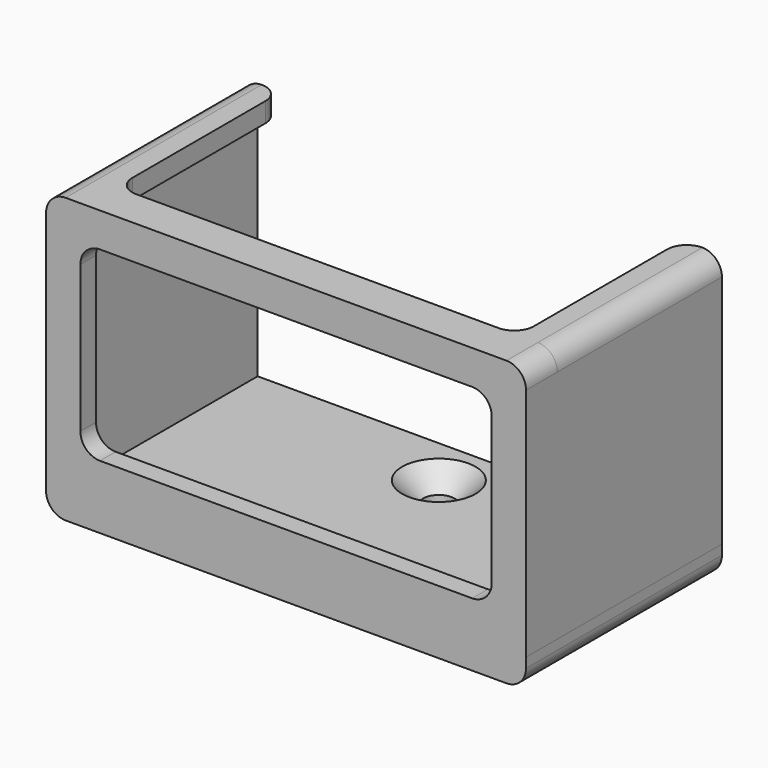
from build123d import *

# Parameters (mm, degrees)
F1_DEPTH        = 24
F2_W            = 4
F2_H            = 21
F3_DEPTH        = 2
F4_W            = 42
F4_H            = 19
F5_DEPTH        = 25
F6_W            = 48.9999982978
F6_H            = 25
F7_DEPTH        = 3
F8_F1_R         = 2
F8_F2_R         = 2
F8_F3_R         = 1.9999
F8_F4_R         = 1.9999
F8_F5_R         = 2
F8_F6_R         = 2
F8_F7_R         = 2
F8_F8_R         = 2
F8_F9_R         = 2
F8_F10_R        = 2
F8_F11_R        = 2
F8_F12_R        = 2
F10_D           = 3.2
F10_CSINK_D     = 7.5
F10_CSINK_ANGLE = 90
F11_R           = 1
F12_SIZE        = 0.5


# Not quite as in the source:
# - a fillet or chamfer is up to 0.001 mm smaller than in the source, because OpenCascade refuses the exact size
# - ends of sketch curves that miss each other by under 0.0002 mm in the source are joined


with BuildPart() as f1:
    # F0 (on Top) → F1 (new body)
    with BuildSketch(Plane.XY):
        Polygon((22.499999217, -11.5), (-22.500000783, -11.5), (-22.499999217, 11.5), (-24.499999217, 11.5), (-24.5000009192, -13.5), (24.4999990808, -13.5), (24.500000783, 11.5), (22.500000783, 11.5), align=None)
    extrude(amount=F1_DEPTH)

    # F2 (on face) → F3 (join)
    with BuildSketch(Plane.XY.offset(24)):
        Polygon((-24.5000009192, -9.5), (-24.5000009192, -13.5), (24.4999993532, -13.5), (24.4999993532, -9.5), (20.500000783, -9.5), (-20.499999217, -9.5), align=None)
        with Locations((-22.499999217, 1)):
            Rectangle(F2_W, F2_H)
        Polygon((20.500000783, -9.5), (24.4999993532, -9.5), (24.500000783, 11.5), (20.500000783, 11.5), align=None)
    extrude(amount=F3_DEPTH)

    # F4 (on face) → F5 (cut)
    with BuildSketch(Plane.XZ.offset(13.5)):
        with Locations((-9.192e-07, 13)):
            Rectangle(F4_W, F4_H)
    extrude(amount=-F5_DEPTH, mode=Mode.SUBTRACT)

    # F6 (on face) → F7 (join)
    with BuildSketch(Plane(origin=(0, 0, 0), x_dir=(1, 0, 0), z_dir=(0, 0, -1))):
        with Locations((-6.81e-08, 1)):
            Rectangle(F6_W, F6_H)
    extrude(amount=F7_DEPTH)

    # F8: fillet of radius 2 on 14 edges, made by hand

    # F8_f1
    f8_f1_edges = [f1.edges().sort_by_distance(p)[0] for p in [
        (20.500000783, 11.5, 25),
    ]]
    fillet(f8_f1_edges, radius=F8_F1_R)

    # F8_f2
    f8_f2_edges = [f1.edges().sort_by_distance(p)[0] for p in [
        (-20.499999217, 11.5, 25),
    ]]
    fillet(f8_f2_edges, radius=F8_F2_R)

    # F8_f3 (radius 2 in the source; OpenCascade refuses exactly that, so slightly less here)
    f8_f3_edges = [f1.edges().sort_by_distance(p)[0] for p in [
        (24.5000000681, 1, 26),
        (24.4999993532, -11.5, 26),
    ]]
    fillet(f8_f3_edges, radius=F8_F3_R)

    # F8_f4 (radius 2 in the source; OpenCascade refuses exactly that, so slightly less here)
    f8_f4_edges = [f1.edges().sort_by_distance(p)[0] for p in [
        (-24.5000009192, -11.5, 26),
    ]]
    fillet(f8_f4_edges, radius=F8_F4_R)

    # F8_f5
    f8_f5_edges = [f1.edges().sort_by_distance(p)[0] for p in [
        (20.500000783, -9.5, 25),
    ]]
    fillet(f8_f5_edges, radius=F8_F5_R)

    # F8_f6
    f8_f6_edges = [f1.edges().sort_by_distance(p)[0] for p in [
        (-21.0000009192, -12.5, 22.5),
    ]]
    fillet(f8_f6_edges, radius=F8_F6_R)

    # F8_f7
    f8_f7_edges = [f1.edges().sort_by_distance(p)[0] for p in [
        (20.9999990808, -12.5, 22.5),
    ]]
    fillet(f8_f7_edges, radius=F8_F7_R)

    # F8_f8
    f8_f8_edges = [f1.edges().sort_by_distance(p)[0] for p in [
        (-21.0000009192, -12.5, 3.5),
    ]]
    fillet(f8_f8_edges, radius=F8_F8_R)

    # F8_f9
    f8_f9_edges = [f1.edges().sort_by_distance(p)[0] for p in [
        (20.9999990808, -12.5, 3.5),
    ]]
    fillet(f8_f9_edges, radius=F8_F9_R)

    # F8_f10
    f8_f10_edges = [f1.edges().sort_by_distance(p)[0] for p in [
        (-20.499999217, -9.5, 25),
    ]]
    fillet(f8_f10_edges, radius=F8_F10_R)

    # F8_f11
    f8_f11_edges = [f1.edges().sort_by_distance(p)[0] for p in [
        (24.4999990808, -1, -3),
    ]]
    fillet(f8_f11_edges, radius=F8_F11_R)

    # F8_f12
    f8_f12_edges = [f1.edges().sort_by_distance(p)[0] for p in [
        (-24.499999217, -1, -3),
    ]]
    fillet(f8_f12_edges, radius=F8_F12_R)

    # F10 (through all)
    with Locations(Plane.XY):
        with Locations((0, 6)):
            CounterSinkHole(F10_D / 2, F10_CSINK_D / 2, counter_sink_angle=F10_CSINK_ANGLE)

    # F11
    f11_edges = [f1.edges().sort_by_distance(p)[0] for p in [
        (-22.500001, -11.5, 12),
        (22.499999, -11.5, 12),
    ]]
    fillet(f11_edges, radius=F11_R)

    # F12
    f12_edges = [f1.edges().sort_by_distance(p)[0] for p in [
        (-22.499999, 11.5, 12),
        (1e-06, 11.5, 0),
        (22.500001, 11.5, 12),
    ]]
    chamfer(f12_edges, length=F12_SIZE)


solid = f1.part
